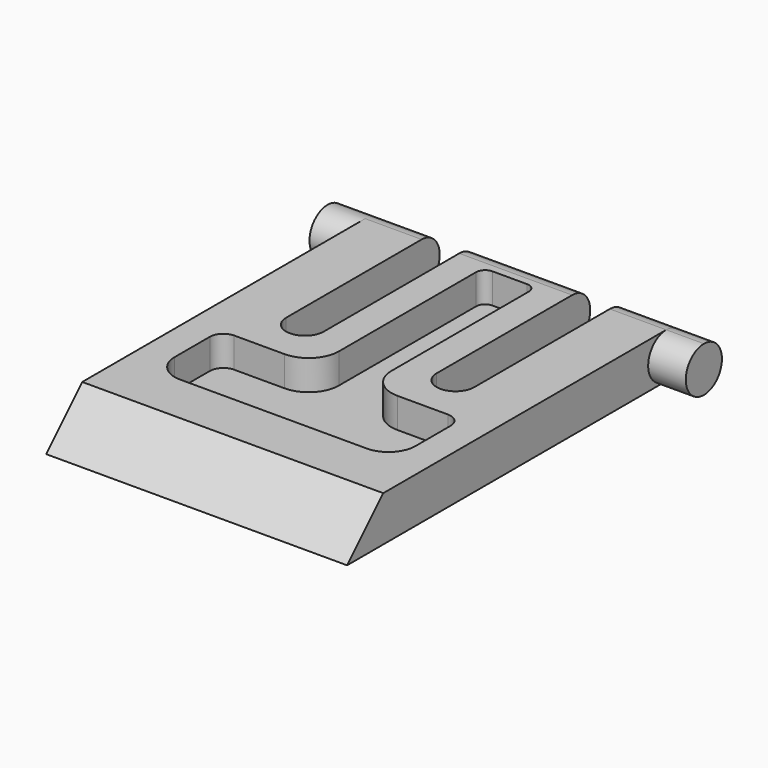
from build123d import *

# Parameters (mm, degrees)
F0_W      = 20
F0_H      = 28
F1_DEPTH  = 3
F3_DEPTH  = 25
F5_DEPTH  = 2
F7_DEPTH  = 32
F9_DEPTH  = 2.5
F10_R     = 1.5
F11_DEPTH = 2.5
F12_DEPTH = 26.07


with BuildPart() as f1:
    # F0 (on Top) → F1 (new body)
    with BuildSketch(Plane.XY):
        with Locations((-10, -14)):
            Rectangle(F0_W, F0_H)
    extrude(amount=F1_DEPTH)

    # F2 (on face) → F3 (cut)
    with BuildSketch(Plane.XY.offset(3)):
        with BuildLine():
            Line((-13.75, -12.75), (-13.75, 0))
            Line((-13.75, 0), (-16.25, 0))
            Line((-16.25, 0), (-16.25, -12.75))
            ThreePointArc((-16.25, -12.75), (-15.883883, -13.633883), (-15, -14))
            ThreePointArc((-15, -14), (-14.116117, -13.633883), (-13.75, -12.75))
        make_face()
        with BuildLine():
            Line((-3.75, -12.75), (-3.75, 0))
            Line((-3.75, 0), (-6.25, 0))
            Line((-6.25, 0), (-6.25, -12.75))
            ThreePointArc((-6.25, -12.75), (-5.883883, -13.633883), (-5, -14))
            ThreePointArc((-5, -14), (-4.116117, -13.633883), (-3.75, -12.75))
        make_face()
    extrude(amount=-F3_DEPTH, mode=Mode.SUBTRACT)

    # F4 (on face) → F5 (cut)
    with BuildSketch(Plane.XY.offset(3)):
        with BuildLine():
            Line((-8.85, -2), (-11.15, -2))
            ThreePointArc((-11.15, -2), (-11.574264, -2.175736), (-11.75, -2.6))
            Line((-11.75, -2.6), (-11.75, -14))
            ThreePointArc((-11.75, -14), (-12.335786, -15.414214), (-13.75, -16))
            Line((-13.75, -16), (-17.1, -16))
            ThreePointArc((-17.1, -16), (-17.736396, -16.263604), (-18, -16.9))
            Line((-18, -16.9), (-18, -19.816884))
            ThreePointArc((-18, -19.816884), (-17.472792, -21.089676), (-16.2, -21.616884))
            Line((-16.2, -21.616884), (-3.8, -21.616884))
            ThreePointArc((-3.8, -21.616884), (-2.527208, -21.089676), (-2, -19.816884))
            Line((-2, -19.816884), (-2, -16.9))
            ThreePointArc((-2, -16.9), (-2.263604, -16.263604), (-2.9, -16))
            Line((-2.9, -16), (-6.25, -16))
            ThreePointArc((-6.25, -16), (-7.664214, -15.414214), (-8.25, -14))
            Line((-8.25, -14), (-8.25, -2.6))
            ThreePointArc((-8.25, -2.6), (-8.425736, -2.175736), (-8.85, -2))
        make_face()
    extrude(amount=-F5_DEPTH, mode=Mode.SUBTRACT)

    # F6 (on face) → F7 (cut)
    with BuildSketch(Plane.YZ):
        Polygon((-28, 3), (-28, 0), (-25, 3), align=None)
    extrude(amount=-F7_DEPTH, mode=Mode.SUBTRACT)

    # F8 (on face) → F9 (join)
    with BuildSketch(Plane.YZ):
        with BuildLine():
            ThreePointArc((-1.5, 0), (-0.43934, 0.43934), (0, 1.5))
            ThreePointArc((0, 1.5), (-0.43934, 2.56066), (-1.5, 3))
            ThreePointArc((-1.5, 3), (-3, 1.5), (-1.5, 0))
        make_face()
    extrude(amount=F9_DEPTH)

    # F10 (on face) → F11 (join)
    with BuildSketch(Plane(origin=(-20, 0, 0), x_dir=(0, -1, 0), z_dir=(-1, 0, 0))):
        with Locations((1.5, 1.5)):
            Circle(F10_R)
    extrude(amount=F11_DEPTH)

    # F12 (cut): faces of the model
    f12_faces = [f1.faces().sort_by_distance(p)[0] for p in [
        (-20, -0.335052, 2.664948),
        (-20, -0.335052, 0.335052),
    ]]
    extrude(f12_faces, amount=-F12_DEPTH, mode=Mode.SUBTRACT)


solid = f1.part
